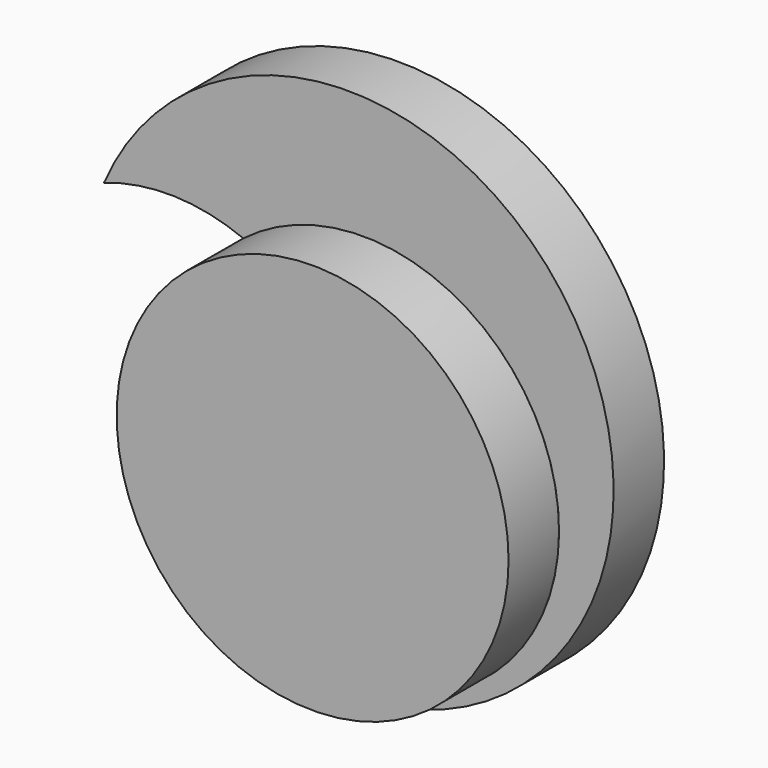
from build123d import *

# Parameters (mm, degrees)
F0_R     = 78.9173451656
F1_DEPTH = 25.4
F3_DEPTH = 25.4


# Not quite as in the source:
# - after a boolean that leaves OpenCascade's solid faulty, fix() repairs it


with BuildPart() as f1:
    # F0 (on Front) → F1 (new body)
    with BuildSketch(Plane.XZ):
        Circle(F0_R)
    extrude(amount=F1_DEPTH)

    # F2 (on face) → F3 (join)
    with BuildSketch(Plane(origin=(0, 0, 0), x_dir=(-1, 0, 0), z_dir=(0, 1, 0))):
        with BuildLine():
            ThreePointArc((78.9173451656, 0), (70.8325817016, 34.7950102381), (48.2347940755, 62.460803777))
            ThreePointArc((48.2347940755, 62.460803777), (0, 0), (29.975245774, -73.0029589042))
            ThreePointArc((29.975245774, -73.0029589042), (65.5496536419, -43.9453100502), (78.9173451656, 0))
        make_face()
    extrude(amount=F3_DEPTH)

    add(f1.part.fix(), mode=Mode.REPLACE)


with BuildPart() as f3:
    # F2 (on face) → F3, piece 2 (new body)
    with BuildSketch(Plane(origin=(0, 0, 0), x_dir=(-1, 0, 0), z_dir=(0, 1, 0))):
        with BuildLine():
            ThreePointArc((48.2347940755, 62.460803777), (76.1521808182, 68.348354975), (104.3385465947, 63.924270215))
            ThreePointArc((104.3385465947, 63.924270215), (-91.6791379898, 64.9839546859), (40.4312930076, -79.8293376001))
            ThreePointArc((40.4312930076, -79.8293376001), (35.0680398169, -76.6232810344), (29.975245774, -73.0029589042))
            ThreePointArc((29.975245774, -73.0029589042), (-78.2100398495, 10.5421551272), (48.2347940755, 62.460803777))
        make_face()
    extrude(amount=F3_DEPTH)


solid = Compound([f1.part, f3.part])
